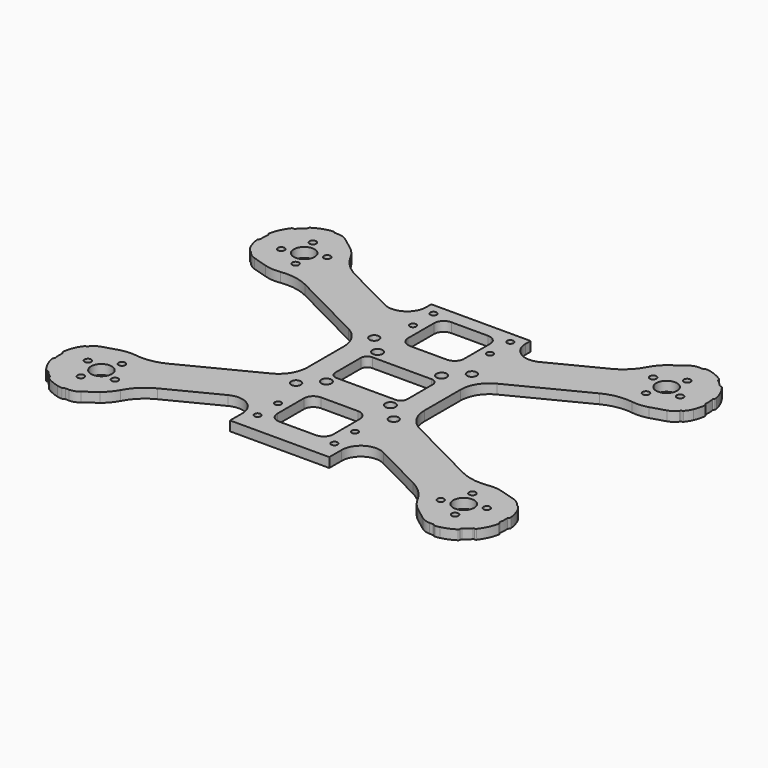
from build123d import *

# Parameters (mm, degrees)
F0_R     = 1.05
F0_R_2   = 3.25
F0_R_3   = 1
F0_R_4   = 1.5
F0_R_5   = 1.6
F1_DEPTH = 3


# Not quite as in the source:
# - ends of sketch curves that miss each other by under 0.0002 mm in the source are joined


with BuildPart() as f1:
    # F0 (on Top) → F1 (new body)
    with BuildSketch(Plane.XY):
        with BuildLine():
            ThreePointArc((46.4257955549, 44.9605572345), (43.6889069418, 41.2736926328), (39.9649518407, 38.5874893127))
            Line((39.9649518407, 38.5874893127), (24.223943, 30.567044))
            ThreePointArc((24.223943, 30.567044), (18.3650084468, 30.7972431149), (15.5, 35.913084))
            Line((15.5, 35.913084), (15.5, 37.849621))
            Line((15.5, 37.849621), (-15.5, 37.849621))
            Line((-15.5, 37.849621), (-15.5, 35.913084))
            ThreePointArc((-15.5, 35.913084), (-18.3650084468, 30.7972431149), (-24.2239426539, 30.5670446793))
            Line((-24.2239426539, 30.5670446793), (-39.964952, 38.587489))
            ThreePointArc((-39.964952, 38.587489), (-43.6889074587, 41.2736921562), (-46.4257963376, 44.9605568221))
            ThreePointArc((-46.4257963376, 44.9605568221), (-47.8412510132, 47.0521350086), (-49.679126909, 48.7843081208))
            Line((-49.679126909, 48.7843081208), (-53.403715, 51.590987))
            ThreePointArc((-53.403715, 51.590987), (-54.7708925567, 52.3205380312), (-56.2957850053, 52.5964397722))
            ThreePointArc((-56.2957850053, 52.5964397722), (-56.8477538199, 52.5976389412), (-57.3992759929, 52.5754058853))
            ThreePointArc((-57.3992759929, 52.5754058853), (-57.6302408222, 52.6162997426), (-57.8171429696, 52.7580200248))
            ThreePointArc((-57.8171429696, 52.7580200248), (-57.9998076104, 52.8978654948), (-58.2257550059, 52.9411191382))
            ThreePointArc((-58.2257550059, 52.9411191382), (-58.9913274624, 52.8712186526), (-59.7466559378, 52.7281587404))
            ThreePointArc((-59.7466559378, 52.7281587404), (-61.9046314452, 52.0141405353), (-63.9122237311, 50.9481885826))
            ThreePointArc((-63.9122237311, 50.9481885826), (-64.0898030922, 50.7490988416), (-64.1397293174, 50.487032974))
            ThreePointArc((-64.1397293174, 50.487032974), (-64.182663849, 50.239741958), (-64.3403513513, 50.044470474))
            ThreePointArc((-64.3403513513, 50.044470474), (-65.3826728437, 49.184605246), (-66.330110227, 48.2211922012))
            ThreePointArc((-66.330110227, 48.2211922012), (-66.5383820678, 48.0811242621), (-66.7884739164, 48.0599054899))
            ThreePointArc((-66.7884739164, 48.0599054899), (-67.0538939677, 48.033009949), (-67.2677032546, 47.8734581975))
            ThreePointArc((-67.2677032546, 47.8734581975), (-68.8351551967, 45.3053463797), (-69.7949041067, 42.4538580231))
            ThreePointArc((-69.7949041067, 42.4538580231), (-69.779693762, 42.1875130415), (-69.6296882841, 41.9669016651))
            ThreePointArc((-69.6296882841, 41.9669016651), (-69.4851871167, 41.761680533), (-69.4586109976, 41.5121009996))
            ThreePointArc((-69.4586109976, 41.5121009996), (-69.5876268783, 40.1670520881), (-69.5763304203, 38.815877035))
            ThreePointArc((-69.5763304203, 38.815877035), (-69.6245575553, 38.5695628337), (-69.78639582, 38.3777167459))
            ThreePointArc((-69.78639582, 38.3777167459), (-69.95505781, 38.1710187171), (-69.9934237569, 37.9070130307))
            ThreePointArc((-69.9934237569, 37.9070130307), (-69.6483334446, 36.1371984868), (-69.070461699, 34.4291601248))
            ThreePointArc((-69.070461699, 34.4291601248), (-68.4933598251, 33.2998249125), (-67.7450383479, 32.2758817007))
            ThreePointArc((-67.7450383479, 32.2758817007), (-67.6002509223, 32.1602384984), (-67.4232910933, 32.1052661913))
            ThreePointArc((-67.4232910933, 32.1052661913), (-67.2295067465, 32.0409543473), (-67.0775887362, 31.9045381937))
            ThreePointArc((-67.0775887362, 31.9045381937), (-67.0069908485, 31.8093298441), (-66.9355277871, 31.7147691624))
            ThreePointArc((-66.9355277871, 31.7147691624), (-65.8160094345, 30.6432758364), (-64.4221829832, 29.966026055))
            Line((-64.4221829832, 29.966026055), (-59.962275, 28.602495))
            ThreePointArc((-59.962275, 28.602495), (-57.4806403901, 28.1337681646), (-54.9565339623, 28.218039739))
            ThreePointArc((-54.9565339623, 28.218039739), (-50.3650954963, 28.170934243), (-46.0030259532, 26.7371020918))
            Line((-46.0030259532, 26.7371020918), (-23.164086, 15.100081))
            ThreePointArc((-23.164086, 15.100081), (-19.5762386701, 11.7835093261), (-18.25, 7.081022))
            Line((-18.25, 7.081022), (-18.25, -7.081023))
            ThreePointArc((-18.25, -7.081023), (-19.5762385515, -11.7835101326), (-23.1640856071, -15.1000817711))
            Line((-23.1640856071, -15.1000817711), (-46.003026, -26.737102))
            ThreePointArc((-46.003026, -26.737102), (-50.3650953429, -28.1709352176), (-54.9565340246, -28.2180401705))
            ThreePointArc((-54.9565340246, -28.2180401705), (-57.4806403901, -28.1337681646), (-59.9622748805, -28.6024953909))
            Line((-59.9622748805, -28.6024953909), (-64.422183, -29.966026))
            ThreePointArc((-64.422183, -29.966026), (-65.8160094345, -30.6432758364), (-66.9355280409, -31.7147689688))
            ThreePointArc((-66.9355280409, -31.7147689688), (-67.0069908485, -31.8093298441), (-67.077588794, -31.9045381513))
            ThreePointArc((-67.077588794, -31.9045381513), (-67.2295067465, -32.0409543473), (-67.4232910074, -32.1052669356))
            ThreePointArc((-67.4232910074, -32.1052669356), (-67.6002505368, -32.160239294), (-67.7450377077, -32.2758822514))
            ThreePointArc((-67.7450377077, -32.2758822514), (-68.4933593843, -33.2998251963), (-69.0704619858, -34.4291600059))
            ThreePointArc((-69.0704619858, -34.4291600059), (-69.6483334446, -36.1371984868), (-69.9934235802, -37.9070130531))
            ThreePointArc((-69.9934235802, -37.9070130531), (-69.95505781, -38.1710187171), (-69.7863958459, -38.3777167824))
            ThreePointArc((-69.7863958459, -38.3777167824), (-69.6245575553, -38.5695628337), (-69.5763303963, -38.8158770365))
            ThreePointArc((-69.5763303963, -38.8158770365), (-69.5876268783, -40.1670520881), (-69.4586107305, -41.5121009599))
            ThreePointArc((-69.4586107305, -41.5121009599), (-69.4851871167, -41.761680533), (-69.6296886278, -41.9669012601))
            ThreePointArc((-69.6296886278, -41.9669012601), (-69.779693762, -42.1875130415), (-69.7949042373, -42.4538580513))
            ThreePointArc((-69.7949042373, -42.4538580513), (-68.8351551967, -45.3053463797), (-67.2677031588, -47.8734581232))
            ThreePointArc((-67.2677031588, -47.8734581232), (-67.0538939677, -48.033009949), (-66.7884739178, -48.0599054818))
            ThreePointArc((-66.7884739178, -48.0599054818), (-66.5383820678, -48.0811242621), (-66.3301103349, -48.2211922967))
            ThreePointArc((-66.3301103349, -48.2211922967), (-65.3826726242, -49.1846054471), (-64.3403508151, -50.0444707505))
            ThreePointArc((-64.3403508151, -50.0444707505), (-64.1826637261, -50.2397422292), (-64.1397286826, -50.487033026))
            ThreePointArc((-64.1397286826, -50.487033026), (-64.0898030922, -50.7490988416), (-63.9122237022, -50.9481885379))
            ThreePointArc((-63.9122237022, -50.9481885379), (-61.9046314452, -52.0141405353), (-59.7466559766, -52.7281589023))
            ThreePointArc((-59.7466559766, -52.7281589023), (-58.9913274624, -52.8712186526), (-58.2257549945, -52.9411188719))
            ThreePointArc((-58.2257549945, -52.9411188719), (-57.9998079637, -52.8978656531), (-57.8171436298, -52.7580204852))
            ThreePointArc((-57.8171436298, -52.7580204852), (-57.630241177, -52.6162998976), (-57.3992759979, -52.5754059655))
            ThreePointArc((-57.3992759979, -52.5754059655), (-56.8477538199, -52.5976389412), (-56.2957849995, -52.5964400215))
            ThreePointArc((-56.2957849995, -52.5964400215), (-54.7708925567, -52.3205380312), (-53.4037155364, -51.5909862881))
            Line((-53.4037155364, -51.5909862881), (-49.679127, -48.784308))
            ThreePointArc((-49.679127, -48.784308), (-47.8412510132, -47.0521350086), (-46.4257959378, -44.9605570328))
            ThreePointArc((-46.4257959378, -44.9605570328), (-43.6889074587, -41.2736921562), (-39.9649520468, -38.5874889082))
            Line((-39.9649520468, -38.5874889082), (-24.223943, -30.567045))
            ThreePointArc((-24.223943, -30.567045), (-18.3650086404, -30.7972429963), (-15.5, -35.913084))
            Line((-15.5, -35.913084), (-15.5, -40.742757))
            Line((-15.5, -40.742757), (15.5, -40.742757))
            Line((15.5, -40.742757), (15.5, -35.913084))
            ThreePointArc((15.5, -35.913084), (18.3650086404, -30.7972429963), (24.2239430584, -30.5670448854))
            Line((24.2239430584, -30.5670448854), (39.964952, -38.587489))
            ThreePointArc((39.964952, -38.587489), (43.6889069418, -41.2736926328), (46.4257955549, -44.9605572345))
            ThreePointArc((46.4257955549, -44.9605572345), (47.8412510132, -47.0521350086), (49.679126909, -48.7843081208))
            Line((49.679126909, -48.7843081208), (53.403715, -51.590987))
            ThreePointArc((53.403715, -51.590987), (54.7708919339, -52.3205381623), (56.2957840053, -52.5964397722))
            ThreePointArc((56.2957840053, -52.5964397722), (56.8477533201, -52.5976389507), (57.3992759929, -52.5754058853))
            ThreePointArc((57.3992759929, -52.5754058853), (57.6302409242, -52.6163002242), (57.8171428602, -52.7580211143))
            ThreePointArc((57.8171428602, -52.7580211143), (57.9998077084, -52.8978659868), (58.2257550041, -52.9411190953))
            ThreePointArc((58.2257550041, -52.9411190953), (58.9913274624, -52.8712186526), (59.7466559378, -52.7281587404))
            ThreePointArc((59.7466559378, -52.7281587404), (61.9046310587, -52.0141407005), (63.9122230244, -50.9481890379))
            ThreePointArc((63.9122230244, -50.9481890379), (64.0898020741, -50.7490988782), (64.1397283241, -50.4870330554))
            ThreePointArc((64.1397283241, -50.4870330554), (64.1826637261, -50.2397422292), (64.3403508729, -50.0444708285))
            ThreePointArc((64.3403508729, -50.0444708285), (65.3826726242, -49.1846054471), (66.330110227, -48.2211922012))
            ThreePointArc((66.330110227, -48.2211922012), (66.5383820678, -48.0811242621), (66.7884739164, -48.0599054899))
            ThreePointArc((66.7884739164, -48.0599054899), (67.0538939677, -48.033009949), (67.2677032546, -47.8734581975))
            ThreePointArc((67.2677032546, -47.8734581975), (68.8351551967, -45.3053463797), (69.7949041067, -42.4538580231))
            ThreePointArc((69.7949041067, -42.4538580231), (69.779693762, -42.1875130415), (69.6296882841, -41.9669016651))
            ThreePointArc((69.6296882841, -41.9669016651), (69.485186225, -41.761680821), (69.4586100193, -41.5121008542))
            ThreePointArc((69.4586100193, -41.5121008542), (69.5876268796, -40.167052058), (69.5763304166, -38.8158769748))
            ThreePointArc((69.5763304166, -38.8158769748), (69.6245573919, -38.5695631744), (69.7863951541, -38.3777172176))
            ThreePointArc((69.7863951541, -38.3777172176), (69.955057671, -38.1710190332), (69.9934237412, -37.9070129063))
            ThreePointArc((69.9934237412, -37.9070129063), (69.6483333794, -36.1371982411), (69.0704615523, -34.429159771))
            ThreePointArc((69.0704615523, -34.429159771), (68.4933585552, -33.299825474), (67.7450372789, -32.2758826204))
            ThreePointArc((67.7450372789, -32.2758826204), (67.600250098, -32.1602390613), (67.4232899926, -32.1052670644))
            ThreePointArc((67.4232899926, -32.1052670644), (67.229506317, -32.0409540979), (67.0775887362, -31.9045381937))
            ThreePointArc((67.0775887362, -31.9045381937), (67.0069906668, -31.8093296013), (66.9355274192, -31.7147686802))
            ThreePointArc((66.9355274192, -31.7147686802), (65.816008827, -30.6432761094), (64.4221828977, -29.9660263346))
            Line((64.4221828977, -29.9660263346), (59.962274, -28.602495))
            ThreePointArc((59.962274, -28.602495), (57.4806399133, -28.133768128), (54.9565339623, -28.218039739))
            ThreePointArc((54.9565339623, -28.218039739), (50.3650949033, -28.1709351449), (46.0030247548, -26.7371024812))
            Line((46.0030247548, -26.7371024812), (23.164085, -15.100081))
            ThreePointArc((23.164085, -15.100081), (19.5762383188, -11.7835097527), (18.25, -7.081023))
            Line((18.25, -7.081023), (18.25, 7.081022))
            ThreePointArc((18.25, 7.081022), (19.5762384374, 11.7835089463), (23.1640852177, 15.1000805727))
            Line((23.1640852177, 15.1000805727), (46.003025, 26.737102))
            ThreePointArc((46.003025, 26.737102), (50.3650950568, 28.1709341703), (54.9565338832, 28.218039191))
            ThreePointArc((54.9565338832, 28.218039191), (57.4806399133, 28.133768128), (59.962273966, 28.6024951113))
            Line((59.962273966, 28.6024951113), (64.422183, 29.966026))
            ThreePointArc((64.422183, 29.966026), (65.816008827, 30.6432761094), (66.9355270409, 31.7147689688))
            ThreePointArc((66.9355270409, 31.7147689688), (67.0069906668, 31.8093296013), (67.077588794, 31.9045381513))
            ThreePointArc((67.077588794, 31.9045381513), (67.229506317, 32.0409540979), (67.4232900205, 32.1052668218))
            ThreePointArc((67.4232900205, 32.1052668218), (67.6002504835, 32.1602382657), (67.7450382021, 32.2758818261))
            ThreePointArc((67.7450382021, 32.2758818261), (68.493358996, 33.2998251902), (69.0704613396, 34.4291598592))
            ThreePointArc((69.0704613396, 34.4291598592), (69.6483333794, 36.1371982411), (69.9934235644, 37.9070129287))
            ThreePointArc((69.9934235644, 37.9070129287), (69.955057671, 38.1710190332), (69.78639518, 38.3777172541))
            ThreePointArc((69.78639518, 38.3777172541), (69.6245573919, 38.5695631744), (69.5763303927, 38.8158769763))
            ThreePointArc((69.5763303927, 38.8158769763), (69.5876268796, 40.167052058), (69.4586107305, 41.5121009599))
            ThreePointArc((69.4586107305, 41.5121009599), (69.485186225, 41.761680821), (69.6296882092, 41.9669017534))
            ThreePointArc((69.6296882092, 41.9669017534), (69.779693762, 42.1875130415), (69.7949042373, 42.4538580513))
            ThreePointArc((69.7949042373, 42.4538580513), (68.8351551967, 45.3053463797), (67.2677031588, 47.8734581232))
            ThreePointArc((67.2677031588, 47.8734581232), (67.0538939677, 48.033009949), (66.7884739178, 48.0599054818))
            ThreePointArc((66.7884739178, 48.0599054818), (66.5383820678, 48.0811242621), (66.3301103349, 48.2211922967))
            ThreePointArc((66.3301103349, 48.2211922967), (65.3826728437, 49.184605246), (64.3403512935, 50.044470396))
            ThreePointArc((64.3403512935, 50.044470396), (64.182663849, 50.239741958), (64.1397286826, 50.487033026))
            ThreePointArc((64.1397286826, 50.487033026), (64.0898020741, 50.7490988782), (63.9122227022, 50.9481885379))
            ThreePointArc((63.9122227022, 50.9481885379), (61.9046310587, 52.0141407005), (59.7466559766, 52.7281589023))
            ThreePointArc((59.7466559766, 52.7281589023), (58.9913274624, 52.8712186526), (58.2257549945, 52.9411188719))
            ThreePointArc((58.2257549945, 52.9411188719), (57.9998073551, 52.8978658285), (57.8171425404, 52.7580203757))
            ThreePointArc((57.8171425404, 52.7580203757), (57.6302405695, 52.6163000692), (57.3992759941, 52.5754059042))
            ThreePointArc((57.3992759941, 52.5754059042), (56.8477533201, 52.5976389507), (56.295784, 52.5964399981))
            ThreePointArc((56.295784, 52.5964399981), (54.7708919339, 52.3205381623), (53.4037151742, 51.5909867688))
            Line((53.4037151742, 51.5909867688), (49.679127, 48.784308))
            ThreePointArc((49.679127, 48.784308), (47.8412510132, 47.0521350086), (46.4257955549, 44.9605572345))
        make_face()
        with Locations((-58.454102, -45.306339)):
            Circle(F0_R, mode=Mode.SUBTRACT)
        with Locations((-50.893661, -41.454102)):
            Circle(F0_R, mode=Mode.SUBTRACT)
        with Locations((-62.306339, -37.745898)):
            Circle(F0_R, mode=Mode.SUBTRACT)
        with Locations((-56.6, -39.6)):
            Circle(F0_R_2, mode=Mode.SUBTRACT)
        with Locations((-54.745898, -33.893661)):
            Circle(F0_R, mode=Mode.SUBTRACT)
        with Locations((-12, -34.349621)):
            Circle(F0_R_3, mode=Mode.SUBTRACT)
        with Locations((-12, -26.349621)):
            Circle(F0_R_3, mode=Mode.SUBTRACT)
        with BuildLine():
            ThreePointArc((-5.75, -33.742757), (-7.8713203436, -32.8640773436), (-8.75, -30.742757))
            Line((-8.75, -30.742757), (-8.75, -20.378187))
            ThreePointArc((-8.75, -20.378187), (-7.8713203436, -18.2568666564), (-5.75, -17.378187))
            Line((-5.75, -17.378187), (5.75, -17.378187))
            ThreePointArc((5.75, -17.378187), (7.8713203436, -18.2568666564), (8.75, -20.378187))
            Line((8.75, -20.378187), (8.75, -30.742757))
            ThreePointArc((8.75, -30.742757), (7.8713203436, -32.8640773436), (5.75, -33.742757))
            Line((5.75, -33.742757), (-5.75, -33.742757))
        make_face(mode=Mode.SUBTRACT)
        with Locations((-15.25, -15.25)):
            Circle(F0_R_4, mode=Mode.SUBTRACT)
        with Locations((-10, -10)):
            Circle(F0_R_5, mode=Mode.SUBTRACT)
        with Locations((12, -34.349621)):
            Circle(F0_R_3, mode=Mode.SUBTRACT)
        with Locations((50.893661, -41.454102)):
            Circle(F0_R, mode=Mode.SUBTRACT)
        with Locations((58.454102, -45.306339)):
            Circle(F0_R, mode=Mode.SUBTRACT)
        with Locations((56.6, -39.6)):
            Circle(F0_R_2, mode=Mode.SUBTRACT)
        with Locations((54.745898, -33.893661)):
            Circle(F0_R, mode=Mode.SUBTRACT)
        with Locations((62.306339, -37.745898)):
            Circle(F0_R, mode=Mode.SUBTRACT)
        with Locations((12, -26.349621)):
            Circle(F0_R_3, mode=Mode.SUBTRACT)
        with Locations((15.25, -15.25)):
            Circle(F0_R_4, mode=Mode.SUBTRACT)
        with Locations((10, -10)):
            Circle(F0_R_5, mode=Mode.SUBTRACT)
        with BuildLine():
            Line((-9.25, 7), (9.25, 7))
            ThreePointArc((9.25, 7), (10.6642135624, 6.4142135624), (11.25, 5))
            Line((11.25, 5), (11.25, -5))
            ThreePointArc((11.25, -5), (10.6642135624, -6.4142135624), (9.25, -7))
            Line((9.25, -7), (-9.25, -7))
            ThreePointArc((-9.25, -7), (-10.6642135624, -6.4142135624), (-11.25, -5))
            Line((-11.25, -5), (-11.25, 5))
            ThreePointArc((-11.25, 5), (-10.6642135624, 6.4142135624), (-9.25, 7))
        make_face(mode=Mode.SUBTRACT)
        with Locations((-10, 10)):
            Circle(F0_R_5, mode=Mode.SUBTRACT)
        with Locations((-15.25, 15.25)):
            Circle(F0_R_4, mode=Mode.SUBTRACT)
        with Locations((-12, 26.349621)):
            Circle(F0_R_3, mode=Mode.SUBTRACT)
        with BuildLine():
            Line((8.75, 30.499261), (8.75, 20.378187))
            ThreePointArc((8.75, 20.378187), (7.8713203436, 18.2568666564), (5.75, 17.378187))
            Line((5.75, 17.378187), (-5.75, 17.378187))
            ThreePointArc((-5.75, 17.378187), (-7.8713203436, 18.2568666564), (-8.75, 20.378187))
            Line((-8.75, 20.378187), (-8.75, 30.499261))
            ThreePointArc((-8.75, 30.499261), (-7.8713203436, 32.6205813436), (-5.75, 33.499261))
            Line((-5.75, 33.499261), (5.75, 33.499261))
            ThreePointArc((5.75, 33.499261), (7.8713203436, 32.6205813436), (8.75, 30.499261))
        make_face(mode=Mode.SUBTRACT)
        with Locations((-62.306339, 37.745898)):
            Circle(F0_R, mode=Mode.SUBTRACT)
        with Locations((-54.745898, 33.893661)):
            Circle(F0_R, mode=Mode.SUBTRACT)
        with Locations((-56.6, 39.6)):
            Circle(F0_R_2, mode=Mode.SUBTRACT)
        with Locations((-58.454102, 45.306339)):
            Circle(F0_R, mode=Mode.SUBTRACT)
        with Locations((-50.893661, 41.454102)):
            Circle(F0_R, mode=Mode.SUBTRACT)
        with Locations((-12, 34.349621)):
            Circle(F0_R_3, mode=Mode.SUBTRACT)
        with Locations((10, 10)):
            Circle(F0_R_5, mode=Mode.SUBTRACT)
        with Locations((15.25, 15.25)):
            Circle(F0_R_4, mode=Mode.SUBTRACT)
        with Locations((12, 26.349621)):
            Circle(F0_R_3, mode=Mode.SUBTRACT)
        with Locations((12, 34.349621)):
            Circle(F0_R_3, mode=Mode.SUBTRACT)
        with Locations((54.745898, 33.893661)):
            Circle(F0_R, mode=Mode.SUBTRACT)
        with Locations((56.6, 39.6)):
            Circle(F0_R_2, mode=Mode.SUBTRACT)
        with Locations((62.306339, 37.745898)):
            Circle(F0_R, mode=Mode.SUBTRACT)
        with Locations((50.893661, 41.454102)):
            Circle(F0_R, mode=Mode.SUBTRACT)
        with Locations((58.454102, 45.306339)):
            Circle(F0_R, mode=Mode.SUBTRACT)
    extrude(amount=F1_DEPTH)


solid = f1.part
